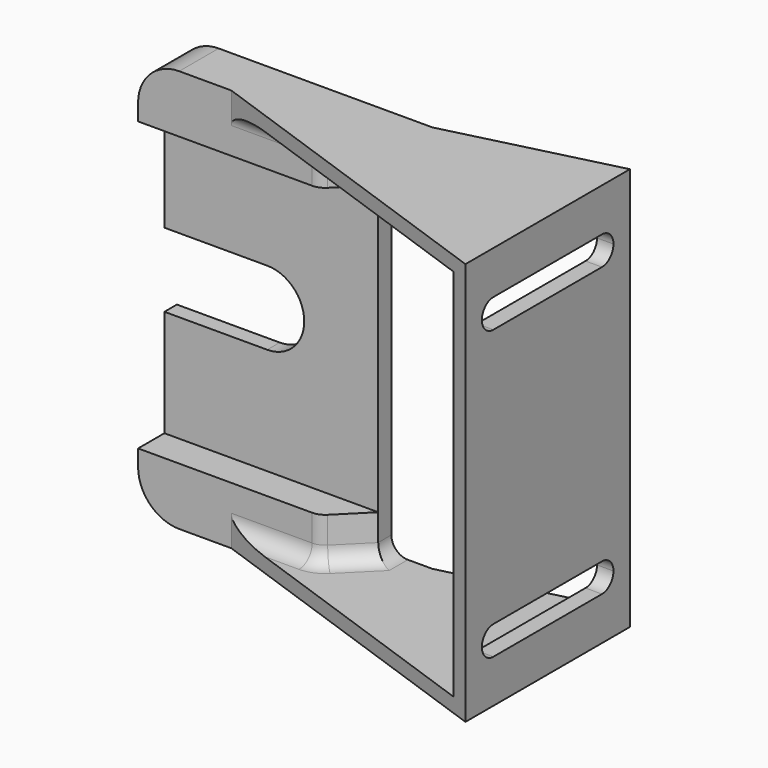
from build123d import *

# Parameters (mm, degrees)
F1_DEPTH  = 49
F3_DEPTH  = 8.001
F4_W      = 18
F4_H      = 45.5
F4_W_2    = 5
F5_DEPTH  = 25
F7_DEPTH  = 2
F8_W      = 33.7460841984
F8_H      = 45.5
F9_DEPTH  = 18.001
F11_DEPTH = 0.1
F12_W     = 26
F12_H     = 1.75
F12_H_2   = 5.25
F13_DEPTH = 4
F14_SIZE  = 4
F15_R     = 2
F16_R     = 5


# Not quite as in the source:
# - a feature names something its author has since deleted; it is built from what else it names


with BuildPart() as f1:
    # F0 (on Top) → F1 (new body)
    with BuildSketch(Plane.XY):
        Polygon((31, 2), (0, 2), (0, 0), (51, -18), (51, 2), align=None)
        Polygon((51, 7), (31, 2), (51, 2), align=None)
    extrude(amount=F1_DEPTH)

    # F2 (on face) → F3 (cut, through all)
    with BuildSketch(Plane(origin=(0, 2, 0), x_dir=(-1, 0, 0), z_dir=(0, 1, 0))):
        with BuildLine():
            Line((0, 29), (-12.5, 29))
            ThreePointArc((-12.5, 29), (-17, 24.5), (-12.5, 20))
            Line((-12.5, 20), (0, 20))
            Line((0, 20), (0, 29))
        make_face()
    extrude(amount=-F3_DEPTH, mode=Mode.SUBTRACT)

    # F4 (on face) → F5 (cut, symmetric)
    with BuildSketch(Plane(origin=(0, 2, 0), x_dir=(-1, 0, 0), z_dir=(0, 1, 0))):
        with Locations((-40, 24.5)):
            Rectangle(F4_W, F4_H)
        with Locations((-28.5, 24.5)):
            Rectangle(F4_W_2, F4_H)
    extrude(amount=F5_DEPTH, both=True, mode=Mode.SUBTRACT)

    # F6 (on face) → F7 (cut, through all)
    with BuildSketch(Plane.YZ.offset(51)):
        with BuildLine():
            ThreePointArc((2.75, 40.25), (1, 42), (2.75, 43.75))
            Line((2.75, 43.75), (-13.75, 43.75))
            ThreePointArc((-13.75, 43.75), (-12.5125631329, 43.2374368671), (-12, 42))
            ThreePointArc((-12, 42), (-12.5125631329, 40.7625631329), (-13.75, 40.25))
            Line((-13.75, 40.25), (2.75, 40.25))
        make_face()
        with BuildLine():
            ThreePointArc((-12, 42), (-12.5125631329, 43.2374368671), (-13.75, 43.75))
            ThreePointArc((-13.75, 43.75), (-15.5, 42), (-13.75, 40.25))
            ThreePointArc((-13.75, 40.25), (-12.5125631329, 40.7625631329), (-12, 42))
        make_face()
        with BuildLine():
            ThreePointArc((2.75, 40.25), (3.9874368671, 40.7625631329), (4.5, 42))
            ThreePointArc((4.5, 42), (3.9874368671, 43.2374368671), (2.75, 43.75))
            ThreePointArc((2.75, 43.75), (1, 42), (2.75, 40.25))
        make_face()
        with BuildLine():
            ThreePointArc((2.75, 5.25), (1, 7), (2.75, 8.75))
            Line((2.75, 8.75), (-13.75, 8.75))
            ThreePointArc((-13.75, 8.75), (-12.5125631329, 8.2374368671), (-12, 7))
            ThreePointArc((-12, 7), (-12.5125631329, 5.7625631329), (-13.75, 5.25))
            Line((-13.75, 5.25), (2.75, 5.25))
        make_face()
        with BuildLine():
            ThreePointArc((-12, 7), (-12.5125631329, 8.2374368671), (-13.75, 8.75))
            ThreePointArc((-13.75, 8.75), (-15.5, 7), (-13.75, 5.25))
            ThreePointArc((-13.75, 5.25), (-12.5125631329, 5.7625631329), (-12, 7))
        make_face()
        with BuildLine():
            ThreePointArc((4.5, 7), (3.9874368671, 8.2374368671), (2.75, 8.75))
            ThreePointArc((2.75, 8.75), (1, 7), (2.75, 5.25))
            ThreePointArc((2.75, 5.25), (3.9874368671, 5.7625631329), (4.5, 7))
        make_face()
    extrude(amount=-F7_DEPTH, mode=Mode.SUBTRACT)

    # F8 (on Front) → F9 (cut, through all)
    with BuildSketch(Plane.XZ):
        with Locations((14.1801619902, 24.5)):
            Rectangle(F8_W, F8_H)
    extrude(amount=F9_DEPTH, mode=Mode.SUBTRACT)

    # F10 (on face) → F11 (cut)
    with BuildSketch(Plane(origin=(0, 2, 0), x_dir=(-1, 0, 0), z_dir=(0, 1, 0))):
        with BuildLine():
            ThreePointArc((-10.3159670332, 16.7), (-6.0462930408, 19.6051387676), (-4.4, 24.5))
            ThreePointArc((-4.4, 24.5), (-6.0462930408, 29.3948612324), (-10.3159670332, 32.3))
            ThreePointArc((-10.3159670332, 32.3), (-20.6, 24.5), (-10.3159670332, 16.7))
        make_face()
        with BuildLine():
            ThreePointArc((-10.3159670332, 32.3), (-6.0462930408, 29.3948612324), (-4.4, 24.5))
            ThreePointArc((-4.4, 24.5), (-6.0462930408, 19.6051387676), (-10.3159670332, 16.7))
            Line((-10.3159670332, 16.7), (0, 16.4))
            Line((0, 16.4), (0, 32.6))
            Line((0, 32.6), (-10.3159670332, 32.3))
        make_face()
    extrude(amount=-F11_DEPTH, mode=Mode.SUBTRACT)

    # F12 (on face) → F13 (join)
    with BuildSketch(Plane.XZ):
        with Locations((13, 48.125)):
            Rectangle(F12_W, F12_H)
        with Locations((13, 0.875)):
            Rectangle(F12_W, F12_H)
        with Locations((13, 44.625)):
            Rectangle(F12_W, F12_H_2)
        with Locations((13, 4.375)):
            Rectangle(F12_W, F12_H_2)
    extrude(amount=F13_DEPTH)

    # F14
    f14_edges = [f1.edges().sort_by_distance(p)[0] for p in [
        (26, -4, 4.375),
        (26, -4, 44.625),
    ]]
    chamfer(f14_edges, length=F14_SIZE)

    # F15
    f15_edges = [f1.edges().sort_by_distance(p)[0] for p in [
        (16.666667, -4, 1.75),
        (16.666667, -4, 47.25),
        (24, -2, 47.25),
        (24, -2, 1.75),
        (22, -4, 4.375),
        (22, -4, 44.625),
        (26, 1, 1.75),
        (26, 1, 47.25),
    ]]
    fillet(f15_edges, radius=F15_R)

    # F16
    f16_edges = [f1.edges().sort_by_distance(p)[0] for p in [
        (0, -1, 49),
        (0, -1, 0),
    ]]
    fillet(f16_edges, radius=F16_R)


solid = f1.part
